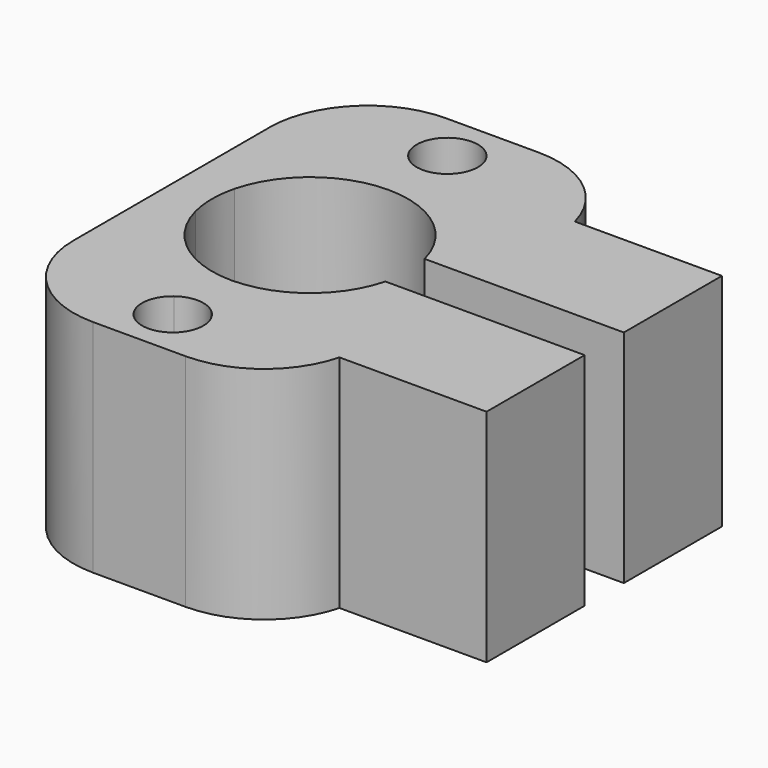
from build123d import *

# Parameters (mm, degrees)
F0_W        = 12
F0_H        = 10
F1_DEPTH    = 18
F2_T1_DEPTH = 56.7298334621
F2_T3_DEPTH = 58


# Not quite as in the source:
# - a fillet or chamfer that OpenCascade refuses, or shapes differently, is made with other operations: its cross-section is extruded or revolved along the edge and cut away or added


with BuildPart() as f1:
    # F0 (on Top) → F1 (new body)
    with BuildSketch(Plane.XY):
        with BuildLine():
            ThreePointArc((14.4251908534, 16.4576590359), (22.1711575458, 22.4576590359), (29.9171242382, 16.4576590359))
            Line((29.9171242382, 16.4576590359), (34.1711575458, 16.4576590359))
            Line((34.1711575458, 16.4576590359), (34.1711575458, 26.4576590359))
            Line((34.1711575458, 26.4576590359), (23.6711575458, 26.4576590359))
            ThreePointArc((23.6711575458, 26.4576590359), (22.1711575458, 25.9576590359), (20.6711575458, 26.4576590359))
            Line((20.6711575458, 26.4576590359), (10.8711575458, 26.4576590359))
            Line((10.8711575458, 26.4576590359), (10.8711575458, 16.4576590359))
            Line((10.8711575458, 16.4576590359), (14.4251908534, 16.4576590359))
        make_face()
        with BuildLine():
            Line((34.1711575458, 12.4576590359), (29.9171242382, 12.4576590359))
            ThreePointArc((29.9171242382, 12.4576590359), (22.1711575458, 6.4576590359), (14.4251908534, 12.4576590359))
            Line((14.4251908534, 12.4576590359), (10.8711575458, 12.4576590359))
            Line((10.8711575458, 12.4576590359), (10.8711575458, 2.4576590359))
            Line((10.8711575458, 2.4576590359), (20.6711575458, 2.4576590359))
            ThreePointArc((20.6711575458, 2.4576590359), (22.1711575458, 2.9576590359), (23.6711575458, 2.4576590359))
            Line((23.6711575458, 2.4576590359), (34.1711575458, 2.4576590359))
            Line((34.1711575458, 2.4576590359), (34.1711575458, 12.4576590359))
        make_face()
        with BuildLine():
            ThreePointArc((14.4251908534, 12.4576590359), (14.1711575458, 14.4576590359), (14.4251908534, 16.4576590359))
            Line((14.4251908534, 16.4576590359), (10.8711575458, 16.4576590359))
            Line((10.8711575458, 16.4576590359), (10.8711575458, 12.4576590359))
            Line((10.8711575458, 12.4576590359), (14.4251908534, 12.4576590359))
        make_face()
        with Locations((40.1711575458, 21.4576590359)):
            Rectangle(F0_W, F0_H)
        with Locations((40.1711575458, 7.4576590359)):
            Rectangle(F0_W, F0_H)
        with BuildLine():
            Line((23.6711575458, 26.4576590359), (34.1711575458, 26.4576590359))
            Line((34.1711575458, 26.4576590359), (34.1711575458, 32.4576590359))
            Line((34.1711575458, 32.4576590359), (10.8711575458, 32.4576590359))
            Line((10.8711575458, 32.4576590359), (10.8711575458, 26.4576590359))
            Line((10.8711575458, 26.4576590359), (20.6711575458, 26.4576590359))
            ThreePointArc((20.6711575458, 26.4576590359), (21.0531235571, 30.6937270134), (24.6711575458, 28.4576590359))
            ThreePointArc((24.6711575458, 28.4576590359), (24.4072255233, 27.3396250472), (23.6711575458, 26.4576590359))
        make_face()
        with BuildLine():
            Line((34.1711575458, -3.5423409641), (34.1711575458, 2.4576590359))
            Line((34.1711575458, 2.4576590359), (23.6711575458, 2.4576590359))
            ThreePointArc((23.6711575458, 2.4576590359), (24.4072255233, 1.5756930247), (24.6711575458, 0.4576590359))
            ThreePointArc((24.6711575458, 0.4576590359), (21.0531235571, -1.7784089416), (20.6711575458, 2.4576590359))
            Line((20.6711575458, 2.4576590359), (10.8711575458, 2.4576590359))
            Line((10.8711575458, 2.4576590359), (10.8711575458, -3.5423409641))
            Line((10.8711575458, -3.5423409641), (34.1711575458, -3.5423409641))
        make_face()
    extrude(amount=F1_DEPTH)

    # F2: fillet of radius 8 on 4 edges, made by hand

    # F2_s2 → F2_t1 (cut)
    with BuildSketch(Plane.XY.offset(-19.364916731)):
        with BuildLine():
            ThreePointArc((34.1711575458, 26.4576590359), (31.324170339, 30.7822143563), (26.4251908534, 32.4576590359))
            Line((26.4251908534, 32.4576590359), (34.1711575458, 32.4576590359))
            Line((34.1711575458, 32.4576590359), (34.1711575458, 26.4576590359))
        make_face()
        with BuildLine():
            ThreePointArc((26.4251908534, -3.5423409641), (31.324170339, -1.8668962844), (34.1711575458, 2.4576590359))
            Line((34.1711575458, 2.4576590359), (34.1711575458, -3.5423409641))
            Line((34.1711575458, -3.5423409641), (26.4251908534, -3.5423409641))
        make_face()
    extrude(amount=F2_T1_DEPTH, mode=Mode.SUBTRACT)

    # F2_s4 → F2_t3 (cut)
    with BuildSketch(Plane.XY.offset(-20)):
        with BuildLine():
            ThreePointArc((10.8711575458, 4.4576590359), (13.2143032963, -1.1991952136), (18.8711575458, -3.5423409641))
            Line((18.8711575458, -3.5423409641), (10.8711575458, -3.5423409641))
            Line((10.8711575458, -3.5423409641), (10.8711575458, 4.4576590359))
        make_face()
        with BuildLine():
            ThreePointArc((18.8711575458, 32.4576590359), (13.2143032963, 30.1145132854), (10.8711575458, 24.4576590359))
            Line((10.8711575458, 24.4576590359), (10.8711575458, 32.4576590359))
            Line((10.8711575458, 32.4576590359), (18.8711575458, 32.4576590359))
        make_face()
    extrude(amount=F2_T3_DEPTH, mode=Mode.SUBTRACT)


solid = f1.part
